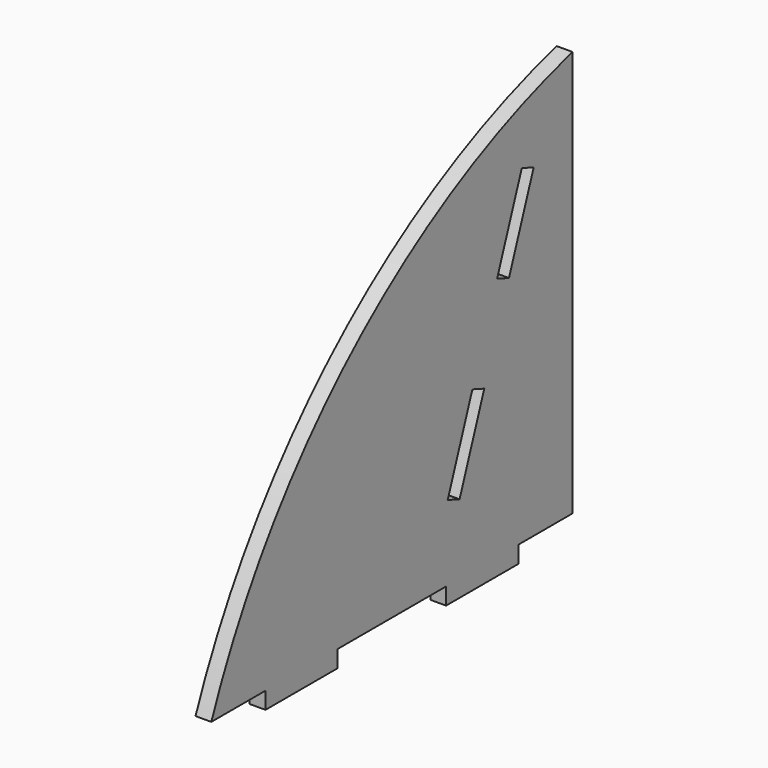
from build123d import *

# Parameters (mm, degrees)
F0_W     = 101.6
F0_H     = 19.05
F1_DEPTH = 17.78


# Not quite as in the source:
# - a feature names something its author has since deleted; it is built from what else it names


with BuildPart() as f1:
    # F0 (on Right) → F1 (new body)
    with BuildSketch(Plane.YZ):
        with BuildLine():
            ThreePointArc((508, 457.2), (375.1962383216, 406.7634952275), (254, 332.6544408126))
            Line((254, 332.6544408126), (254, 0))
            Line((254, 0), (330.2, 0))
            Line((330.2, 0), (431.8, 0))
            Line((431.8, 0), (508, 0))
            Line((508, 0), (508, 457.2))
        make_face()
        Polygon((349.8489306504, 132.4179212181), (367.2235539314, 180.154306354), (383.9312887289, 174.0731882056), (349.182042167, 78.6004179338), (332.4743073695, 84.6815360821), align=None, mode=Mode.SUBTRACT)
        Polygon((401.9728004932, 275.6270766258), (419.3474237742, 323.3634617617), (436.7220470551, 371.0998468977), (453.4297818527, 365.0187287493), (418.6805352908, 269.5459584775), align=None, mode=Mode.SUBTRACT)
        Polygon((127, 0), (76.2, 0), (76.2, -19.05), (177.8, -19.05), (177.8, 0), align=None)
        with BuildLine():
            ThreePointArc((254, 332.6544408126), (103.8213611206, 184.0253886947), (0, 0))
            Line((0, 0), (76.2, 0))
            Line((76.2, 0), (127, 0))
            Line((127, 0), (177.8, 0))
            Line((177.8, 0), (254, 0))
            Line((254, 0), (254, 332.6544408126))
        make_face()
        with Locations((381, -9.525)):
            Rectangle(F0_W, F0_H)
    extrude(amount=F1_DEPTH)


solid = f1.part
